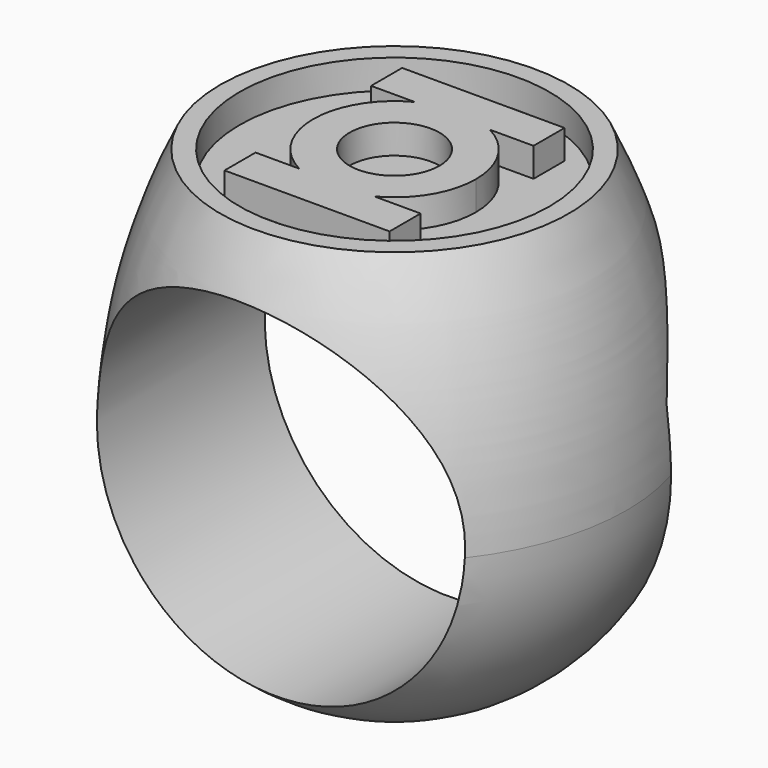
from build123d import *

# Parameters (mm, degrees)
F2_R     = 9.5
F3_DEPTH = 12.7
F4_R     = 8
F5_DEPTH = 1.5
F7_DEPTH = 12.7


# Not quite as in the source:
# - ends of sketch curves that miss each other by under 0.0002 mm in the source are joined
# - a feature names something its author has since deleted; it is built from what else it names


with BuildPart() as f1:
    # F0 (on Front) → F1 (revolve)
    with BuildSketch(Plane.XZ):
        with BuildLine():
            ThreePointArc((-12, -12.5), (-8.4852813742, -20.9852813742), (0, -24.5))
            Line((0, -24.5), (0, -12.5))
            Line((0, -12.5), (-12, -12.5))
        make_face()
        with BuildLine():
            Line((-12, -12.5), (0, -12.5))
            Line((0, -12.5), (0, 0))
            Line((0, 0), (-9, 0))
            ThreePointArc((-9, 0), (-11.177394056, -6.0874254266), (-12, -12.5))
        make_face()
    revolve(axis=Axis((0, 0, -12.25), (0, 0, 1)))

    # F2 (on Front) → F3 (cut, symmetric)
    with BuildSketch(Plane.XZ):
        with Locations((0, -12.25)):
            Circle(F2_R)
    extrude(amount=F3_DEPTH, both=True, mode=Mode.SUBTRACT)

    # F4 (on Top) → F5 (cut)
    with BuildSketch(Plane.XY):
        Circle(F4_R)
        with BuildLine():
            ThreePointArc((-1.9356951783, -3.7273427769), (-3.58956263, -2.1806054493), (-4.2, 0))
            ThreePointArc((-4.2, 0), (-3.58956263, 2.1806054493), (-1.9356951783, 3.7273427769))
            Line((-1.9356951783, 3.7273427769), (-4.191, 3.7254119238))
            Line((-4.191, 3.7254119238), (-4.191, 5.729))
            Line((-4.191, 5.729), (0, 5.729))
            Line((0, 5.729), (4.191, 5.7290075347))
            Line((4.191, 5.7290075347), (4.191, 3.7289706524))
            Line((4.191, 3.7289706524), (1.9325573402, 3.7289706524))
            ThreePointArc((1.9325573402, 3.7289706524), (3.5886446487, 2.1821158506), (4.2, 0))
            ThreePointArc((4.2, 0), (3.58956263, -2.1806054493), (1.9356951783, -3.7273427769))
            Line((1.9356951783, -3.7273427769), (4.3272348121, -3.7273427769))
            Line((4.3272348121, -3.7273427769), (4.3272348121, -5.7290102))
            Line((4.3272348121, -5.7290102), (0, -5.7290102))
            Line((0, -5.7290102), (-4.191, -5.7290102))
            Line((-4.191, -5.7290102), (-4.191, -3.7273427769))
            Line((-4.191, -3.7273427769), (-1.9356951783, -3.7273427769))
        make_face(mode=Mode.SUBTRACT)
        with BuildLine():
            ThreePointArc((-2.32, 0), (0, -2.32), (2.32, 0))
            ThreePointArc((2.32, 0), (0, 2.32), (-2.32, 0))
        make_face()
    extrude(amount=-F5_DEPTH, mode=Mode.SUBTRACT)

    # F6 (on Right) → F7 (cut, symmetric)
    with BuildSketch(Plane.YZ):
        with BuildLine():
            Line((3.5, -9.3865861699), (3.5, -26.5))
            Line((3.5, -26.5), (11.7441575179, -26.5))
            Line((11.7441575179, -26.5), (11.7441575179, -12.5))
            Line((11.7441575179, -12.5), (11.7441575179, -2.5))
            Line((11.7441575179, -2.5), (10.2463875179, -2.5))
            ThreePointArc((10.2463875179, -2.5), (6.0394031611, -5.1264769814), (3.5, -9.3865861699))
        make_face()
    extrude(amount=F7_DEPTH, both=True, mode=Mode.SUBTRACT)


solid = f1.part
